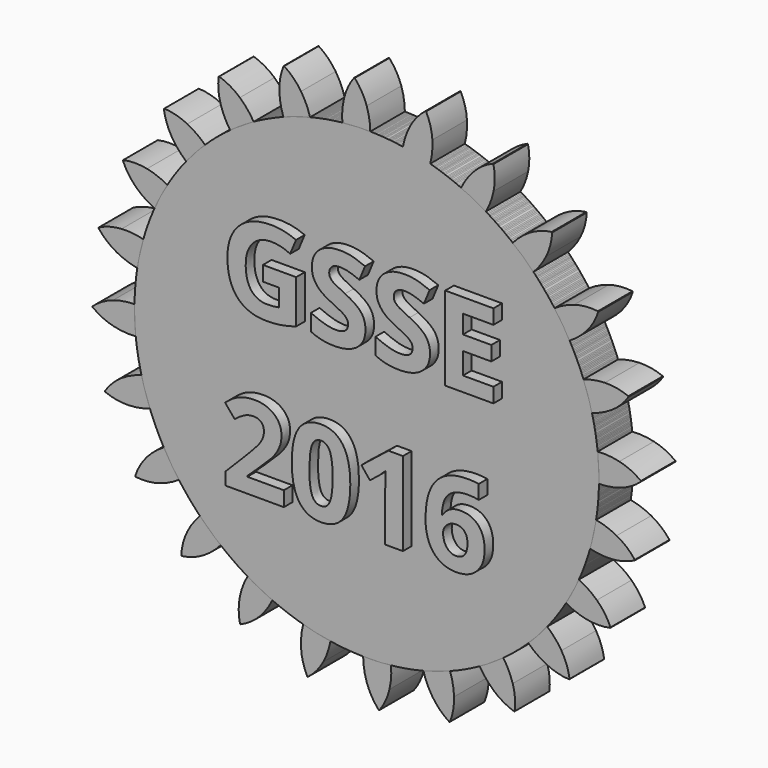
from build123d import *

# Parameters (mm, degrees)
F1_DEPTH     = 5
F2_COUNT     = 24
F2_ANGLE     = 345
F3_TEXT_SIZE = 27.1217021186
F4_DEPTH     = 2.5


# Not quite as in the source:
# - Text() gives the source's letters only with a copy of the font that has no kerning and outlines rounded to 1/6400 em; it was checked with that copy


with BuildPart() as f1:
    # F0 (on Front) → F1 (new body, symmetric)
    with BuildSketch(Plane.XZ):
        with BuildLine():
            ThreePointArc((-5.6379186143, 53.4243363524), (-35.937941059, -39.9300667848), (53.721, 0))
            ThreePointArc((53.721, 0), (38.2776164727, 37.6931017318), (0.8266042082, 53.7146401504))
            ThreePointArc((0.8266042082, 53.7146401504), (-2.4100322928, 53.6669133205), (-5.6379186143, 53.4243363524))
        make_face()
        with BuildLine():
            ThreePointArc((-5.6379186143, 53.4243363524), (-2.4100322928, 53.6669133205), (0.8266042082, 53.7146401504))
            ThreePointArc((0.8266042082, 53.7146401504), (0.605817465, 56.2264076857), (0, 58.674))
            ThreePointArc((0, 58.674), (-1.1413539621, 61.201669581), (-2.7801523292, 63.4391105945))
            ThreePointArc((-2.7801523292, 63.4391105945), (-2.8489441957, 63.440660801), (-2.9173202104, 63.4329507653))
            ThreePointArc((-2.9173202104, 63.4329507653), (-4.3489719806, 61.0576243485), (-5.2591674004, 58.4378253724))
            ThreePointArc((-5.2591674004, 58.4378253724), (-5.6431595864, 55.9457834508), (-5.6379186143, 53.4243363524))
        make_face()
    extrude(amount=F1_DEPTH, both=True)


with BuildPart() as f2_1:
    # F2: instance of F1
    add(f1.part.rotate(Axis((0, 0, 0), (0, -1, 0)), 1 * F2_ANGLE / (F2_COUNT - 1)))


with BuildPart() as f2_2:
    # F2: instance of F1
    add(f1.part.rotate(Axis((0, 0, 0), (0, -1, 0)), 2 * F2_ANGLE / (F2_COUNT - 1)))


with BuildPart() as f2_3:
    # F2: instance of F1
    add(f1.part.rotate(Axis((0, 0, 0), (0, -1, 0)), 3 * F2_ANGLE / (F2_COUNT - 1)))


with BuildPart() as f2_4:
    # F2: instance of F1
    add(f1.part.rotate(Axis((0, 0, 0), (0, -1, 0)), 4 * F2_ANGLE / (F2_COUNT - 1)))


with BuildPart() as f2_5:
    # F2: instance of F1
    add(f1.part.rotate(Axis((0, 0, 0), (0, -1, 0)), 5 * F2_ANGLE / (F2_COUNT - 1)))


with BuildPart() as f2_6:
    # F2: instance of F1
    add(f1.part.rotate(Axis((0, 0, 0), (0, -1, 0)), 6 * F2_ANGLE / (F2_COUNT - 1)))


with BuildPart() as f2_7:
    # F2: instance of F1
    add(f1.part.rotate(Axis((0, 0, 0), (0, -1, 0)), 7 * F2_ANGLE / (F2_COUNT - 1)))


with BuildPart() as f2_8:
    # F2: instance of F1
    add(f1.part.rotate(Axis((0, 0, 0), (0, -1, 0)), 8 * F2_ANGLE / (F2_COUNT - 1)))


with BuildPart() as f2_9:
    # F2: instance of F1
    add(f1.part.rotate(Axis((0, 0, 0), (0, -1, 0)), 9 * F2_ANGLE / (F2_COUNT - 1)))


with BuildPart() as f2_10:
    # F2: instance of F1
    add(f1.part.rotate(Axis((0, 0, 0), (0, -1, 0)), 10 * F2_ANGLE / (F2_COUNT - 1)))


with BuildPart() as f2_11:
    # F2: instance of F1
    add(f1.part.rotate(Axis((0, 0, 0), (0, -1, 0)), 11 * F2_ANGLE / (F2_COUNT - 1)))


with BuildPart() as f2_12:
    # F2: instance of F1
    add(f1.part.rotate(Axis((0, 0, 0), (0, -1, 0)), 12 * F2_ANGLE / (F2_COUNT - 1)))


with BuildPart() as f2_13:
    # F2: instance of F1
    add(f1.part.rotate(Axis((0, 0, 0), (0, -1, 0)), 13 * F2_ANGLE / (F2_COUNT - 1)))


with BuildPart() as f2_14:
    # F2: instance of F1
    add(f1.part.rotate(Axis((0, 0, 0), (0, -1, 0)), 14 * F2_ANGLE / (F2_COUNT - 1)))


with BuildPart() as f2_15:
    # F2: instance of F1
    add(f1.part.rotate(Axis((0, 0, 0), (0, -1, 0)), 15 * F2_ANGLE / (F2_COUNT - 1)))


with BuildPart() as f2_16:
    # F2: instance of F1
    add(f1.part.rotate(Axis((0, 0, 0), (0, -1, 0)), 16 * F2_ANGLE / (F2_COUNT - 1)))


with BuildPart() as f2_17:
    # F2: instance of F1
    add(f1.part.rotate(Axis((0, 0, 0), (0, -1, 0)), 17 * F2_ANGLE / (F2_COUNT - 1)))


with BuildPart() as f2_18:
    # F2: instance of F1
    add(f1.part.rotate(Axis((0, 0, 0), (0, -1, 0)), 18 * F2_ANGLE / (F2_COUNT - 1)))


with BuildPart() as f2_19:
    # F2: instance of F1
    add(f1.part.rotate(Axis((0, 0, 0), (0, -1, 0)), 19 * F2_ANGLE / (F2_COUNT - 1)))


with BuildPart() as f2_20:
    # F2: instance of F1
    add(f1.part.rotate(Axis((0, 0, 0), (0, -1, 0)), 20 * F2_ANGLE / (F2_COUNT - 1)))


with BuildPart() as f2_21:
    # F2: instance of F1
    add(f1.part.rotate(Axis((0, 0, 0), (0, -1, 0)), 21 * F2_ANGLE / (F2_COUNT - 1)))


with BuildPart() as f2_22:
    # F2: instance of F1
    add(f1.part.rotate(Axis((0, 0, 0), (0, -1, 0)), 22 * F2_ANGLE / (F2_COUNT - 1)))


with BuildPart() as f2_23:
    # F2: instance of F1
    add(f1.part.rotate(Axis((0, 0, 0), (0, -1, 0)), 23 * F2_ANGLE / (F2_COUNT - 1)))


with BuildPart() as f4:
    # F3 (on face) → F4 (new body)
    with BuildSketch(Plane.XZ.offset(5)):
        with Locations((-31.7914318293, 9.2727001756)):
            Text('GSSE', F3_TEXT_SIZE, font='Open Sans', font_style=FontStyle.BOLD, text_align=(TextAlign.LEFT, TextAlign.BOTTOM))
        with Locations((-31.7914318293, -27.6128147056)):
            Text('2016', F3_TEXT_SIZE, font='Open Sans', font_style=FontStyle.BOLD, text_align=(TextAlign.LEFT, TextAlign.BOTTOM))
    extrude(amount=F4_DEPTH)


solid = Compound([f1.part, f2_1.part, f2_2.part, f2_3.part, f2_4.part, f2_5.part, f2_6.part, f2_7.part, f2_8.part, f2_9.part, f2_10.part, f2_11.part, f2_12.part, f2_13.part, f2_14.part, f2_15.part, f2_16.part, f2_17.part, f2_18.part, f2_19.part, f2_20.part, f2_21.part, f2_22.part, f2_23.part, f4.part])
